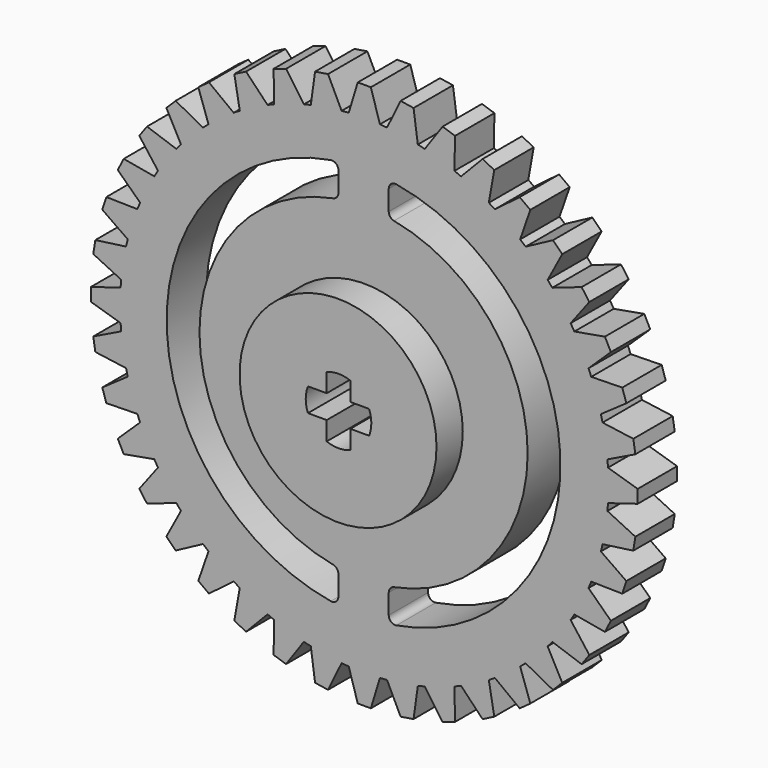
from build123d import *

# Parameters (mm, degrees)
F0_R     = 7.5
F1_DEPTH = 1.875
F2_COUNT = 40
F3_DEPTH = 4.375
F5_DEPTH = 8.751
F7_DEPTH = 13.25


with BuildPart() as f1:
    # F0 (on Front) → F1 (new body, symmetric)
    with BuildSketch(Plane.XZ):
        with BuildLine():
            ThreePointArc((0, 18.6), (0.594128128, 18.5905086474), (1.1876499033, 18.5620442761))
            Line((1.1876499033, 18.5620442761), (0.5, 20.825))
            Line((0.5, 20.825), (0, 20.825))
            Line((0, 20.825), (0, 18.6))
        make_face()
        with BuildLine():
            Line((-0.5, 20.825), (-1.1876499033, 18.5620442761))
            ThreePointArc((-1.1876499033, 18.5620442761), (-0.594128128, 18.5905086474), (0, 18.6))
            Line((0, 18.6), (0, 20.825))
            Line((0, 20.825), (-0.5, 20.825))
        make_face()
        with BuildLine():
            ThreePointArc((-1.1876499033, 18.5620442761), (-12.7253627021, -13.5655867584), (18.6, 0))
            ThreePointArc((18.6, 0), (13.5655867584, 12.7253627021), (1.1876499033, 18.5620442761))
            ThreePointArc((1.1876499033, 18.5620442761), (0.594128128, 18.5905086474), (0, 18.6))
            ThreePointArc((0, 18.6), (-0.594128128, 18.5905086474), (-1.1876499033, 18.5620442761))
        make_face()
        Circle(F0_R, mode=Mode.SUBTRACT)
    extrude(amount=F1_DEPTH, both=True)


with BuildPart() as f2_1:
    # F2: instance of F1
    add(f1.part.rotate(Axis((0, -1.875, 0), (0, -1, 0)), 1 * 360 / F2_COUNT))


with BuildPart() as f2_2:
    # F2: instance of F1
    add(f1.part.rotate(Axis((0, -1.875, 0), (0, -1, 0)), 2 * 360 / F2_COUNT))


with BuildPart() as f2_3:
    # F2: instance of F1
    add(f1.part.rotate(Axis((0, -1.875, 0), (0, -1, 0)), 3 * 360 / F2_COUNT))


with BuildPart() as f2_4:
    # F2: instance of F1
    add(f1.part.rotate(Axis((0, -1.875, 0), (0, -1, 0)), 4 * 360 / F2_COUNT))


with BuildPart() as f2_5:
    # F2: instance of F1
    add(f1.part.rotate(Axis((0, -1.875, 0), (0, -1, 0)), 5 * 360 / F2_COUNT))


with BuildPart() as f2_6:
    # F2: instance of F1
    add(f1.part.rotate(Axis((0, -1.875, 0), (0, -1, 0)), 6 * 360 / F2_COUNT))


with BuildPart() as f2_7:
    # F2: instance of F1
    add(f1.part.rotate(Axis((0, -1.875, 0), (0, -1, 0)), 7 * 360 / F2_COUNT))


with BuildPart() as f2_8:
    # F2: instance of F1
    add(f1.part.rotate(Axis((0, -1.875, 0), (0, -1, 0)), 8 * 360 / F2_COUNT))


with BuildPart() as f2_9:
    # F2: instance of F1
    add(f1.part.rotate(Axis((0, -1.875, 0), (0, -1, 0)), 9 * 360 / F2_COUNT))


with BuildPart() as f2_10:
    # F2: instance of F1
    add(f1.part.rotate(Axis((0, -1.875, 0), (0, -1, 0)), 10 * 360 / F2_COUNT))


with BuildPart() as f2_11:
    # F2: instance of F1
    add(f1.part.rotate(Axis((0, -1.875, 0), (0, -1, 0)), 11 * 360 / F2_COUNT))


with BuildPart() as f2_12:
    # F2: instance of F1
    add(f1.part.rotate(Axis((0, -1.875, 0), (0, -1, 0)), 12 * 360 / F2_COUNT))


with BuildPart() as f2_13:
    # F2: instance of F1
    add(f1.part.rotate(Axis((0, -1.875, 0), (0, -1, 0)), 13 * 360 / F2_COUNT))


with BuildPart() as f2_14:
    # F2: instance of F1
    add(f1.part.rotate(Axis((0, -1.875, 0), (0, -1, 0)), 14 * 360 / F2_COUNT))


with BuildPart() as f2_15:
    # F2: instance of F1
    add(f1.part.rotate(Axis((0, -1.875, 0), (0, -1, 0)), 15 * 360 / F2_COUNT))


with BuildPart() as f2_16:
    # F2: instance of F1
    add(f1.part.rotate(Axis((0, -1.875, 0), (0, -1, 0)), 16 * 360 / F2_COUNT))


with BuildPart() as f2_17:
    # F2: instance of F1
    add(f1.part.rotate(Axis((0, -1.875, 0), (0, -1, 0)), 17 * 360 / F2_COUNT))


with BuildPart() as f2_18:
    # F2: instance of F1
    add(f1.part.rotate(Axis((0, -1.875, 0), (0, -1, 0)), 18 * 360 / F2_COUNT))


with BuildPart() as f2_19:
    # F2: instance of F1
    add(f1.part.rotate(Axis((0, -1.875, 0), (0, -1, 0)), 19 * 360 / F2_COUNT))


with BuildPart() as f2_20:
    # F2: instance of F1
    add(f1.part.rotate(Axis((0, -1.875, 0), (0, -1, 0)), 20 * 360 / F2_COUNT))


with BuildPart() as f2_21:
    # F2: instance of F1
    add(f1.part.rotate(Axis((0, -1.875, 0), (0, -1, 0)), 21 * 360 / F2_COUNT))


with BuildPart() as f2_22:
    # F2: instance of F1
    add(f1.part.rotate(Axis((0, -1.875, 0), (0, -1, 0)), 22 * 360 / F2_COUNT))


with BuildPart() as f2_23:
    # F2: instance of F1
    add(f1.part.rotate(Axis((0, -1.875, 0), (0, -1, 0)), 23 * 360 / F2_COUNT))


with BuildPart() as f2_24:
    # F2: instance of F1
    add(f1.part.rotate(Axis((0, -1.875, 0), (0, -1, 0)), 24 * 360 / F2_COUNT))


with BuildPart() as f2_25:
    # F2: instance of F1
    add(f1.part.rotate(Axis((0, -1.875, 0), (0, -1, 0)), 25 * 360 / F2_COUNT))


with BuildPart() as f2_26:
    # F2: instance of F1
    add(f1.part.rotate(Axis((0, -1.875, 0), (0, -1, 0)), 26 * 360 / F2_COUNT))


with BuildPart() as f2_27:
    # F2: instance of F1
    add(f1.part.rotate(Axis((0, -1.875, 0), (0, -1, 0)), 27 * 360 / F2_COUNT))


with BuildPart() as f2_28:
    # F2: instance of F1
    add(f1.part.rotate(Axis((0, -1.875, 0), (0, -1, 0)), 28 * 360 / F2_COUNT))


with BuildPart() as f2_29:
    # F2: instance of F1
    add(f1.part.rotate(Axis((0, -1.875, 0), (0, -1, 0)), 29 * 360 / F2_COUNT))


with BuildPart() as f2_30:
    # F2: instance of F1
    add(f1.part.rotate(Axis((0, -1.875, 0), (0, -1, 0)), 30 * 360 / F2_COUNT))


with BuildPart() as f2_31:
    # F2: instance of F1
    add(f1.part.rotate(Axis((0, -1.875, 0), (0, -1, 0)), 31 * 360 / F2_COUNT))


with BuildPart() as f2_32:
    # F2: instance of F1
    add(f1.part.rotate(Axis((0, -1.875, 0), (0, -1, 0)), 32 * 360 / F2_COUNT))


with BuildPart() as f2_33:
    # F2: instance of F1
    add(f1.part.rotate(Axis((0, -1.875, 0), (0, -1, 0)), 33 * 360 / F2_COUNT))


with BuildPart() as f2_34:
    # F2: instance of F1
    add(f1.part.rotate(Axis((0, -1.875, 0), (0, -1, 0)), 34 * 360 / F2_COUNT))


with BuildPart() as f2_35:
    # F2: instance of F1
    add(f1.part.rotate(Axis((0, -1.875, 0), (0, -1, 0)), 35 * 360 / F2_COUNT))


with BuildPart() as f2_36:
    # F2: instance of F1
    add(f1.part.rotate(Axis((0, -1.875, 0), (0, -1, 0)), 36 * 360 / F2_COUNT))


with BuildPart() as f2_37:
    # F2: instance of F1
    add(f1.part.rotate(Axis((0, -1.875, 0), (0, -1, 0)), 37 * 360 / F2_COUNT))


with BuildPart() as f2_38:
    # F2: instance of F1
    add(f1.part.rotate(Axis((0, -1.875, 0), (0, -1, 0)), 38 * 360 / F2_COUNT))


with BuildPart() as f2_39:
    # F2: instance of F1
    add(f1.part.rotate(Axis((0, -1.875, 0), (0, -1, 0)), 39 * 360 / F2_COUNT))


with BuildPart() as f1_1:
    add(f1.part)

    add(f2_1.part)  # F3 merges F2_1

    add(f2_2.part)  # F3 merges F2_2

    add(f2_3.part)  # F3 merges F2_3

    add(f2_4.part)  # F3 merges F2_4

    add(f2_5.part)  # F3 merges F2_5

    add(f2_6.part)  # F3 merges F2_6

    add(f2_7.part)  # F3 merges F2_7

    add(f2_8.part)  # F3 merges F2_8

    add(f2_9.part)  # F3 merges F2_9

    add(f2_10.part)  # F3 merges F2_10

    add(f2_11.part)  # F3 merges F2_11

    add(f2_12.part)  # F3 merges F2_12

    add(f2_13.part)  # F3 merges F2_13

    add(f2_14.part)  # F3 merges F2_14

    add(f2_15.part)  # F3 merges F2_15

    add(f2_16.part)  # F3 merges F2_16

    add(f2_17.part)  # F3 merges F2_17

    add(f2_18.part)  # F3 merges F2_18

    add(f2_19.part)  # F3 merges F2_19

    add(f2_20.part)  # F3 merges F2_20

    add(f2_21.part)  # F3 merges F2_21

    add(f2_22.part)  # F3 merges F2_22

    add(f2_23.part)  # F3 merges F2_23

    add(f2_24.part)  # F3 merges F2_24

    add(f2_25.part)  # F3 merges F2_25

    add(f2_26.part)  # F3 merges F2_26

    add(f2_27.part)  # F3 merges F2_27

    add(f2_28.part)  # F3 merges F2_28

    add(f2_29.part)  # F3 merges F2_29

    add(f2_30.part)  # F3 merges F2_30

    add(f2_31.part)  # F3 merges F2_31

    add(f2_32.part)  # F3 merges F2_32

    add(f2_33.part)  # F3 merges F2_33

    add(f2_34.part)  # F3 merges F2_34

    add(f2_35.part)  # F3 merges F2_35

    add(f2_36.part)  # F3 merges F2_36

    add(f2_37.part)  # F3 merges F2_37

    add(f2_38.part)  # F3 merges F2_38

    add(f2_39.part)  # F3 merges F2_39
    # F0 (on Front) → F3 (join, symmetric)
    with BuildSketch(Plane.XZ):
        Circle(F0_R)
    extrude(amount=F3_DEPTH, both=True)

    # F4 (on face) → F5 (cut, through all)
    with BuildSketch(Plane.XZ.offset(4.375)):
        with BuildLine():
            ThreePointArc((2.3675935674, -0.9213311631), (2.493004252, -0.4790757202), (2.5352847075, -0.0213311631))
            ThreePointArc((2.5352847075, -0.0213311631), (2.493004252, 0.4364133941), (2.3675935674, 0.8786688369))
            Line((2.3675935674, 0.8786688369), (0.9362847075, 0.8786688369))
            Line((0.9362847075, 0.8786688369), (0.9362847075, 2.3099776968))
            ThreePointArc((0.9362847075, 2.3099776968), (0.0362847075, 2.4776688369), (-0.8637152925, 2.3099776968))
            Line((-0.8637152925, 2.3099776968), (-0.8637152925, 0.8786688369))
            Line((-0.8637152925, 0.8786688369), (-2.2950241523, 0.8786688369))
            ThreePointArc((-2.2950241523, 0.8786688369), (-2.4627152925, -0.0213311631), (-2.2950241523, -0.9213311631))
            Line((-2.2950241523, -0.9213311631), (-0.8637152925, -0.9213311631))
            Line((-0.8637152925, -0.9213311631), (-0.8637152925, -2.3526400229))
            ThreePointArc((-0.8637152925, -2.3526400229), (0.0362847075, -2.5203311631), (0.9362847075, -2.3526400229))
            Line((0.9362847075, -2.3526400229), (0.9362847075, -0.9213311631))
            Line((0.9362847075, -0.9213311631), (2.3675935674, -0.9213311631))
        make_face()
    extrude(amount=-F5_DEPTH, mode=Mode.SUBTRACT)

    # F6 (on Front) → F7 (cut, symmetric)
    with BuildSketch(Plane.XZ):
        with BuildLine():
            ThreePointArc((-1.9744990182, 14.4548813381), (-2.1517653344, 14.8367752623), (-2.5578708954, 14.9478814701))
            ThreePointArc((-2.5578708954, 14.9478814701), (-15.0567145798, 0.1578775118), (-2.5578708954, -14.6321264464))
            ThreePointArc((-2.5578708954, -14.6321264464), (-2.1517653344, -14.5210202386), (-1.9744990182, -14.1391263145))
            Line((-1.9744990182, -14.1391263145), (-1.9744990182, -12.6153099686))
            ThreePointArc((-1.9744990182, -12.6153099686), (-2.0894692437, -12.2963239615), (-2.3815073091, -12.124033527))
            ThreePointArc((-2.3815073091, -12.124033527), (-12.5567145798, 0.1578775118), (-2.3815073091, 12.4397885507))
            ThreePointArc((-2.3815073091, 12.4397885507), (-2.0894692437, 12.6120789851), (-1.9744990182, 12.9310649922))
            Line((-1.9744990182, 12.9310649922), (-1.9744990182, 14.4548813381))
        make_face()
        with BuildLine():
            Line((1.8610698585, -12.6153099686), (1.8610698585, -14.1391263145))
            ThreePointArc((1.8610698585, -14.1391263145), (2.0383361747, -14.5210202386), (2.4444417357, -14.6321264464))
            ThreePointArc((2.4444417357, -14.6321264464), (14.9432854202, 0.1578775118), (2.4444417357, 14.9478814701))
            ThreePointArc((2.4444417357, 14.9478814701), (2.0383361747, 14.8367752623), (1.8610698585, 14.4548813381))
            Line((1.8610698585, 14.4548813381), (1.8610698585, 12.9310649922))
            ThreePointArc((1.8610698585, 12.9310649922), (1.976040084, 12.6120789851), (2.2680781494, 12.4397885507))
            ThreePointArc((2.2680781494, 12.4397885507), (12.4432854202, 0.1578775118), (2.2680781494, -12.124033527))
            ThreePointArc((2.2680781494, -12.124033527), (1.976040084, -12.2963239615), (1.8610698585, -12.6153099686))
        make_face()
    extrude(amount=F7_DEPTH, both=True, mode=Mode.SUBTRACT)


solid = f1_1.part
